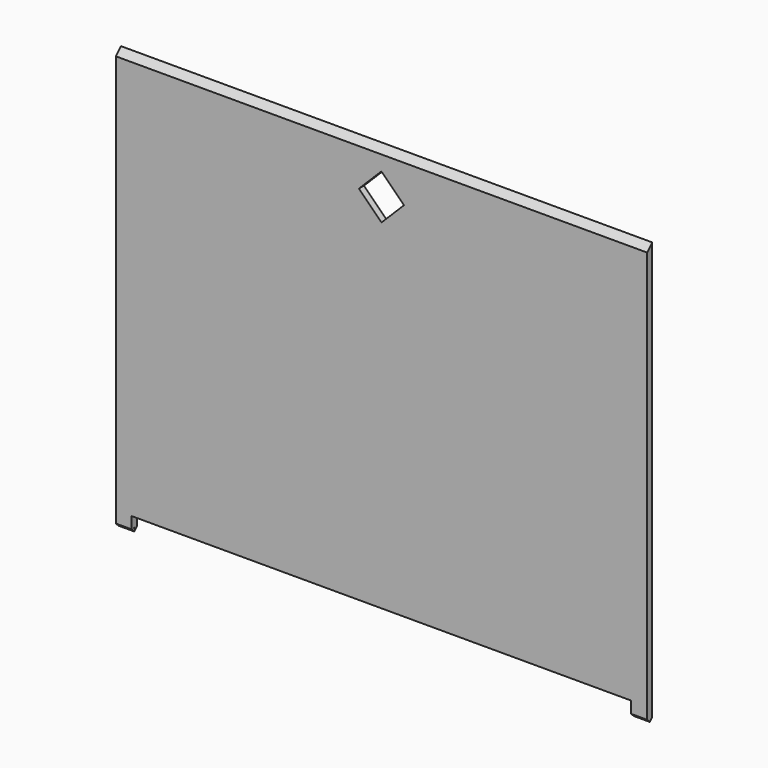
from build123d import *

# Parameters (mm, degrees)
F0_W        = 250
F0_H        = 198.5
F1_DEPTH    = 3
F2_W        = 235
F2_H        = 7.5
F3_DEPTH    = 30
F5_DEPTH    = 300
F6_T1_DEPTH = 17.7867319519
F6_T3_DEPTH = 17.7867319519
F8_DEPTH    = 25
F9_SIZE     = 2.99999
F10_R       = 1.05
F11_DEPTH   = 1.1


# Not quite as in the source:
# - a fillet or chamfer that OpenCascade refuses, or shapes differently, is made with other operations: its cross-section is extruded or revolved along the edge and cut away or added
# - a fillet or chamfer is up to 0.001 mm smaller than in the source, because OpenCascade refuses the exact size


with BuildPart() as f1:
    # F0 (on Front) → F1 (new body)
    with BuildSketch(Plane.XZ):
        Rectangle(F0_W, F0_H)
    extrude(amount=F1_DEPTH)

    # F2 (on face) → F3 (cut)
    with BuildSketch(Plane.XZ.offset(3)):
        with Locations((0, -95.5)):
            Rectangle(F2_W, F2_H)
    extrude(amount=-F3_DEPTH, mode=Mode.SUBTRACT)

    # F4 (on face) → F5 (cut)
    with BuildSketch(Plane.YZ.offset(-117.5)):
        with BuildLine():
            ThreePointArc((-1.25, -97.25), (-1.6767766953, -97.0732233047), (-1.5, -97.5))
            ThreePointArc((-1.5, -97.5), (-1.3232233047, -97.4267766953), (-1.25, -97.25))
        make_face()
    extrude(amount=-F5_DEPTH, mode=Mode.SUBTRACT)

    # F6: chamfer of 2 on 4 edges, made by hand

    # F6_s2 → F6_t1 (cut)
    with BuildSketch(Plane.YZ.offset(-130.1433659759)):
        Polygon((-3, -97.25), (-1, -99.25), (-3, -99.25), align=None)
        Polygon((0, -97.25), (-2, -99.25), (0, -99.25), align=None)
    extrude(amount=F6_T1_DEPTH, mode=Mode.SUBTRACT)

    # F6_s4 → F6_t3 (cut)
    with BuildSketch(Plane.YZ.offset(112.3566340241)):
        Polygon((-3, -97.25), (-1, -99.25), (-3, -99.25), align=None)
        Polygon((0, -97.25), (-2, -99.25), (0, -99.25), align=None)
    extrude(amount=F6_T3_DEPTH, mode=Mode.SUBTRACT)

    # F7 (on face) → F8 (cut)
    with BuildSketch(Plane.XZ.offset(3)):
        Polygon((0, 89.25), (-10.6066017178, 78.6433982822), (0, 68.0367965644), (10.6066017178, 78.6433982822), align=None)
    extrude(amount=-F8_DEPTH, mode=Mode.SUBTRACT)

    # F9 (size 3 in the source; OpenCascade refuses exactly that, so slightly less here)
    f9_edges = [f1.edges().sort_by_distance(p)[0] for p in [
        (0, -3, 99.25),
    ]]
    chamfer(f9_edges, length=F9_SIZE)

    # F10 (on face) → F11 (cut)
    with BuildSketch(Plane(origin=(0, 0, 0), x_dir=(-1, 0, 0), z_dir=(0, 1, 0))):
        with BuildLine():
            Line((-122.45, 93.25), (-123.5, 93.25))
            Line((-123.5, 93.25), (-124.55, 93.25))
            ThreePointArc((-124.55, 93.25), (-123.5, 92.2), (-122.45, 93.25))
        make_face()
        with BuildLine():
            Line((-123.5, 94.3), (-123.5, 93.25))
            Line((-123.5, 93.25), (-122.45, 93.25))
            ThreePointArc((-122.45, 93.25), (-122.7575378798, 93.9924621202), (-123.5, 94.3))
        make_face()
        with BuildLine():
            Line((-124.55, 93.25), (-123.5, 93.25))
            Line((-123.5, 93.25), (-123.5, 94.3))
            ThreePointArc((-123.5, 94.3), (-124.2424621202, 93.9924621202), (-124.55, 93.25))
        make_face()
        with Locations((123.5, 93.25)):
            Circle(F10_R)
    extrude(amount=-F11_DEPTH, mode=Mode.SUBTRACT)


solid = f1.part
